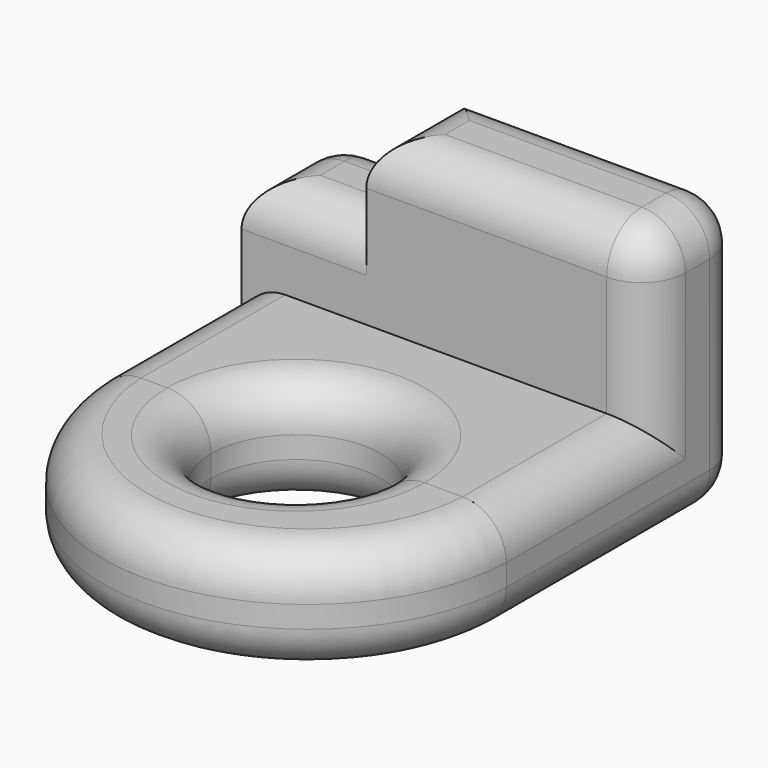
from build123d import *

# Parameters (mm, degrees)
F2_DEPTH = 12.7
F1_W     = 47.5227199495
F1_H     = 34.6339703538
F3_W     = 47.5227199495
F3_H     = 13.6917554773
F4_DEPTH = 19.05
F5_W     = 14.4984591752
F5_H     = 13.6917554773
F6_DEPTH = 8.89
F7_R     = 9.8722552071
F8_DEPTH = 31.751
F10_R    = 5.08
F10_2_R  = 5.08


# Not quite as in the source:
# - a feature of the source that left no trace in its solid (it failed there, or was rolled back) is left out


with BuildPart() as f2:
    # F0 (on Top) → F2 (new body)
    with BuildSketch(Plane.XY):
        with BuildLine():
            Line((24.4325827807, 0), (-23.0901371688, 0))
            ThreePointArc((-23.0901371688, 0), (0.671222806, -22.885776239), (24.4325827807, 0))
        make_face()
    extrude(amount=F2_DEPTH)


with BuildPart() as f2b:
    # F1 (on Top) → F2, piece 2 (new body)
    with BuildSketch(Plane.XY):
        with Locations((0.671222806, 17.3169851769)):
            Rectangle(F1_W, F1_H)
    extrude(amount=F2_DEPTH)

    # F3 (on face) → F4 (join)
    with BuildSketch(Plane.XY.offset(12.7)):
        with Locations((0.671222806, 27.7880926151)):
            Rectangle(F3_W, F3_H)
    extrude(amount=F4_DEPTH)

    # F5 (on face) → F6 (cut)
    with BuildSketch(Plane.XY.offset(31.75)):
        with Locations((-15.8409075812, 27.7880926151)):
            Rectangle(F5_W, F5_H)
    extrude(amount=-F6_DEPTH, mode=Mode.SUBTRACT)


with BuildPart() as f8_tool:
    # F7 (on Top) → F8 (new body, through all)
    with BuildSketch(Plane.XY):
        Circle(F7_R)
    extrude(amount=F8_DEPTH)


with BuildPart() as f2_1:
    add(f2.part)

    # F8: cut by f8_tool
    add(f8_tool.part, mode=Mode.SUBTRACT)

    # F10#2
    f10_2_edges = [f2_1.edges().sort_by_distance(p)[0] for p in [
        (0.671223, -22.885776, 0),
        (0, -9.872255, 0),
        (0, -9.872255, 12.7),
        (0.671223, -22.885776, 12.7),
    ]]
    fillet(f10_2_edges, radius=F10_2_R)


with BuildPart() as f2b_1:
    add(f2b.part)

    # F8: cut by f8_tool
    add(f8_tool.part, mode=Mode.SUBTRACT)

    # F10
    f10_edges = [f2b_1.edges().sort_by_distance(p)[0] for p in [
        (7.920452, 20.942215, 31.75),
        (-15.840908, 20.942215, 22.86),
        (-8.591678, 27.788093, 31.75),
        (7.920452, 34.63397, 31.75),
        (24.432583, 27.788093, 31.75),
        (-15.840908, 34.63397, 22.86),
        (-23.090137, 27.788093, 22.86),
        (-23.090137, 34.63397, 11.43),
        (24.432583, 34.63397, 15.875),
        (24.432583, 20.942215, 22.225),
        (24.432583, 10.471107, 12.7),
        (24.432583, 17.316985, 0),
        (0, 9.872255, 12.7),
        (-23.090137, 10.471107, 12.7),
        (0.671223, 34.63397, 0),
        (0, 9.872255, 0),
        (-23.090137, 17.316985, 0),
    ]]
    fillet(f10_edges, radius=F10_R)


solid = Compound([f2_1.part, f2b_1.part])
